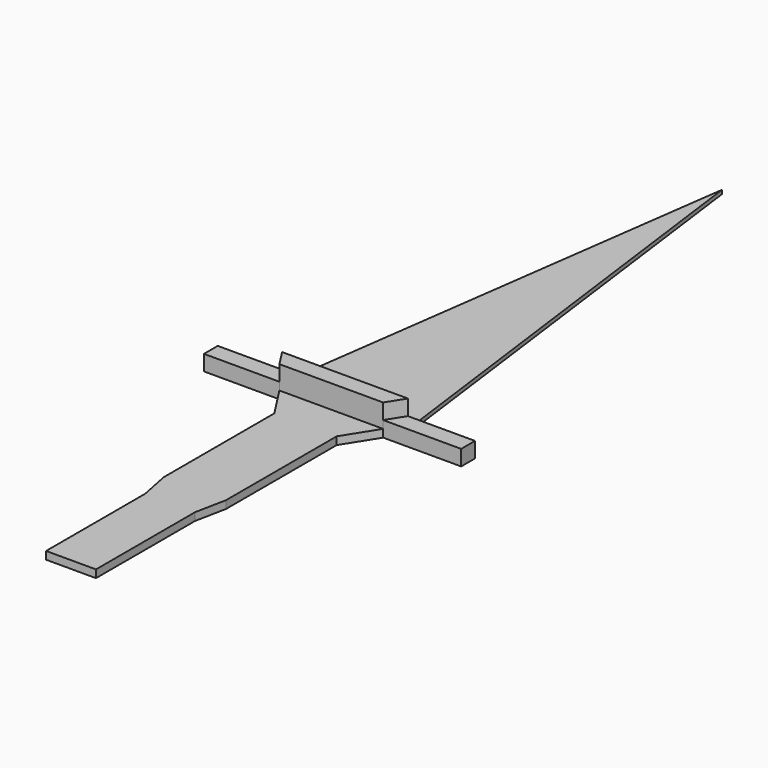
from build123d import *

# Parameters (mm, degrees)
F1_DEPTH = 1.5875
F2_DEPTH = 6.35
F3_DEPTH = 12.7
F0_W     = 25.548312813
F0_H     = 56.7093666971
F4_DEPTH = 3.175


# Not quite as in the source:
# - a length typed as a fraction of an inch, garbled in the dataset ("3 / 203.2 mm" for 3/8 in), is restored


with BuildPart() as f1:
    # F0 (on Top) → F1 (new body)
    with BuildSketch(Plane.XY):
        Polygon((0, 192.5335675478), (0, 0), (25.2136345953, 0), align=None)
        Polygon((-26.3801887631, 0), (0, 0), (0, 192.5335675478), align=None)
    extrude(amount=F1_DEPTH)


with BuildPart() as f2:
    # F0 (on Top) → F2 (new body)
    with BuildSketch(Plane.XY):
        Polygon((52.7516193688, 0), (25.2136345953, 0), (20.757119148, -7.0914621465), (52.7516193688, -7.0914621465), align=None)
    extrude(amount=F2_DEPTH)


with BuildPart() as f2b:
    # F0 (on Top) → F2, piece 2 (new body)
    with BuildSketch(Plane.XY):
        Polygon((-21.8076522841, -7.0914621465), (-26.3801887631, 0), (-52.7603775263, 0), (-52.7603775263, -7.0914621465), align=None)
    extrude(amount=F2_DEPTH)


with BuildPart() as f3:
    # F0 (on Top) → F3 (new body)
    with BuildSketch(Plane.XY):
        Polygon((25.2136345953, 0), (0, 0), (-26.3801887631, 0), (-21.8076522841, -7.0914621465), (20.757119148, -7.0914621465), align=None)
    extrude(amount=F3_DEPTH)

    # F0 (on Top) → F4 (join)
    with BuildSketch(Plane.XY):
        Polygon((12.3582184315, -77.1656398058), (-13.1900943816, -77.1656398058), (-10.6500943816, -89.8656398058), (-10.6500943816, -140.6656398058), (9.8182184315, -140.6656398058), (9.8182184315, -89.8656398058), align=None)
        with Locations((-0.415937975, -48.8109564573)):
            Rectangle(F0_W, F0_H)
        Polygon((20.757119148, -7.0914621465), (-21.8076522841, -7.0914621465), (-13.1900943816, -20.4562731087), (12.3582184315, -20.4562731087), align=None)
    extrude(amount=F4_DEPTH)


solid = Compound([f1.part, f2.part, f2b.part, f3.part])
